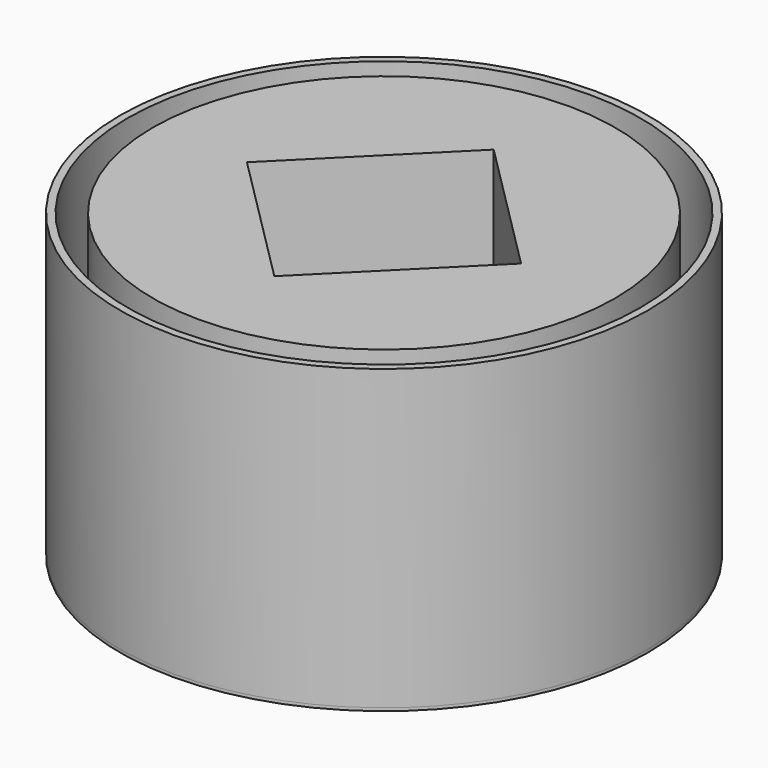
from build123d import *

# Parameters (mm, degrees)
F2_R     = 44.958
F3_DEPTH = 0.508
F4_R     = 39.37
F5_DEPTH = 50.8
F7_DEPTH = 33.02
F8_R     = 44.958
F8_R_2   = 43.688
F9_DEPTH = 50.8


# Not quite as in the source:
# - the program builds the solid bodies; features that only make, move or delete a surface that nothing else refers to are left out


with BuildPart() as f3:
    # F2 (on Top) → F3 (new body)
    with BuildSketch(Plane.XY):
        Circle(F2_R)
    extrude(amount=-F3_DEPTH)

    # F4 (on Top) → F5 (join)
    with BuildSketch(Plane.XY):
        Circle(F4_R)
    extrude(amount=F5_DEPTH)

    # F6 (on face) → F7 (cut)
    with BuildSketch(Plane.XY.offset(50.8)):
        Polygon((23.3486659148, 0), (0, 23.3486659148), (-23.3486659148, 0), (0, -23.3486659148), align=None)
    extrude(amount=-F7_DEPTH, mode=Mode.SUBTRACT)

    # F8 (on Top) → F9 (join)
    with BuildSketch(Plane.XY):
        Circle(F8_R)
        Circle(F8_R_2, mode=Mode.SUBTRACT)
    extrude(amount=F9_DEPTH)


solid = f3.part
